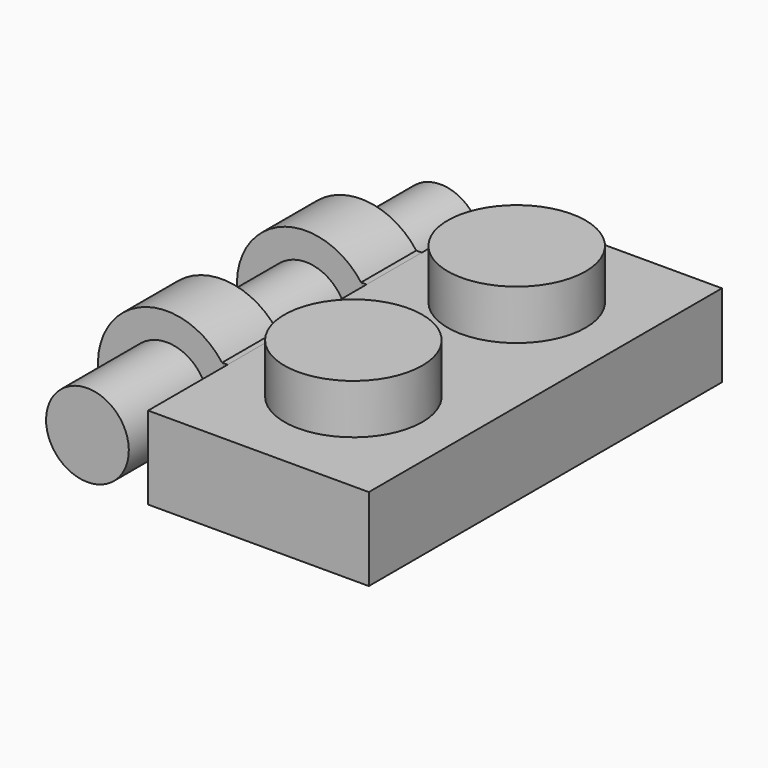
from build123d import *

# Parameters (mm, degrees)
F0_W      = 8
F0_H      = 3
F1_DEPTH  = 16
F2_R      = 2.5
F3_DEPTH  = 1.8
F4_W      = 2.5
F4_H      = 3
F5_DEPTH  = 2.2
F6_W      = 2.5
F6_H      = 1
F6_W_2    = 3.6
F6_H_2    = 1.5
F9_DEPTH  = 2
F10_R     = 1.5
F11_DEPTH = 2


with BuildPart() as f1:
    # F0 (on Front) → F1 (new body)
    with BuildSketch(Plane.XZ):
        with Locations((-4, -1.5)):
            Rectangle(F0_W, F0_H)
    extrude(amount=F1_DEPTH)

    # F2 (on face) → F3 (join)
    with BuildSketch(Plane.XY):
        with Locations((-4, -4.3)):
            Circle(F2_R)
        with Locations((-4, -11.7)):
            Circle(F2_R)
    extrude(amount=F3_DEPTH)

    # F8 (on face) → F9 (cut)
    with BuildSketch(Plane(origin=(0, 0, -3), x_dir=(1, 0, 0), z_dir=(0, 0, -1))):
        Polygon((-6.6, 14.6), (-6.6, 8), (-6.6, 1.4), (-1.4, 1.4), (-1.4, 14.6), align=None)
    extrude(amount=-F9_DEPTH, mode=Mode.SUBTRACT)

    # F10 (on face) → F11 (join)
    with BuildSketch(Plane(origin=(0, 0, -1), x_dir=(1, 0, 0), z_dir=(0, 0, -1))):
        with Locations((-4, 8)):
            Circle(F10_R)
    extrude(amount=F11_DEPTH)


with BuildPart() as f5:
    # F4 (on face) → F5 (new body)
    with BuildSketch(Plane(origin=(-8, 0, 0), x_dir=(0, -1, 0), z_dir=(-1, 0, 0))):
        with Locations((4.85, -1.5)):
            Rectangle(F4_W, F4_H)
    extrude(amount=F5_DEPTH)


with BuildPart() as f5b:
    # F4 (on face) → F5, piece 2 (new body)
    with BuildSketch(Plane(origin=(-8, 0, 0), x_dir=(0, -1, 0), z_dir=(-1, 0, 0))):
        with Locations((11.15, -1.5)):
            Rectangle(F4_W, F4_H)
    extrude(amount=F5_DEPTH)


with BuildPart() as f7:
    # F6 (on face) → F7 (revolve)
    with BuildSketch(Plane(origin=(-10.2, 0, 0), x_dir=(0, -1, 0), z_dir=(-1, 0, 0))):
        with Locations((4.85, -3.5)):
            Rectangle(F6_W, F6_H)
        with Locations((11.15, -3.5)):
            Rectangle(F6_W, F6_H)
        with Locations((14.2, -2.25)):
            Rectangle(F6_W_2, F6_H_2)
        with Locations((11.15, -2.25)):
            Rectangle(F6_W, F6_H_2)
        Polygon((6.1, -3), (9.9, -3), (9.9, -1.5), (0, -1.5), (0, -3), (3.6, -3), align=None)
    revolve(axis=Axis((-10.2, -8, -1.5), (0, -1, 0)))


solid = Compound([f1.part, f5.part, f5b.part, f7.part])
